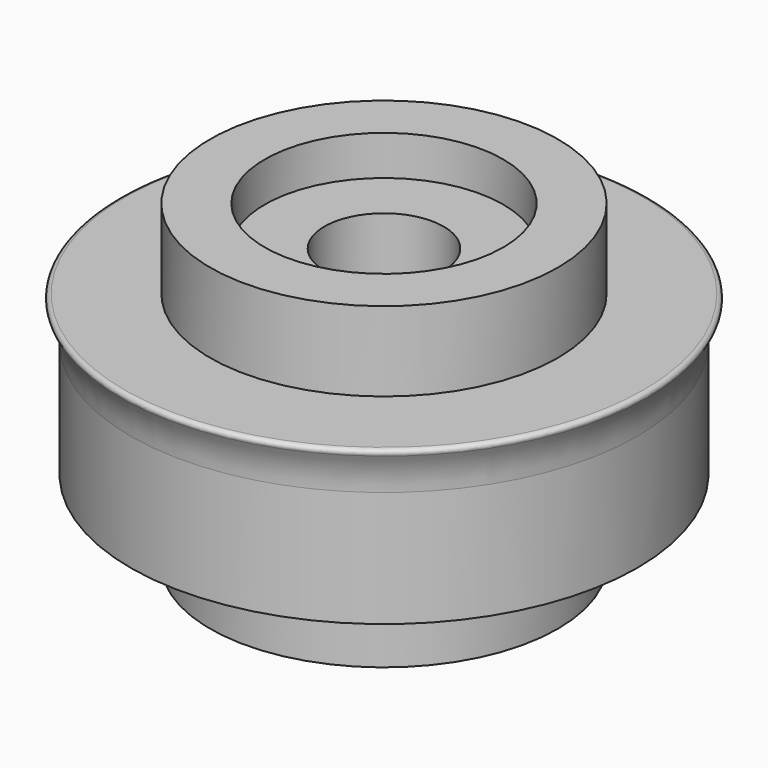
from build123d import *

# Parameters (mm, degrees)
F2_R = 11
F4_R = 0.8


# Not quite as in the source:
# - a fillet or chamfer that OpenCascade refuses, or shapes differently, is made with other operations: its cross-section is extruded or revolved along the edge and cut away or added


with BuildPart() as f1:
    # F0 (on Front) → F1 (revolve)
    with BuildSketch(Plane.XZ):
        Polygon((24, 85.4892928004), (24, 77.4892928004), (12, 77.4892928004), (12, 38.1360072643), (24, 38.1360072643), (24, 21.4892928004), (35, 21.4892928004), (35, 37.4892928004), (51, 37.4892928004), (51, 65.592944622), (51, 69.4892928004), (35, 69.4892928004), (35, 85.4892928004), align=None)
        Polygon((53.7719889283, 69.4892928004), (51, 69.4892928004), (51, 65.592944622), align=None)
    revolve(axis=Axis((0, 0, 48.0438946244), (0, 0, 1)))

    # F2
    f2_edges = [f1.edges().sort_by_distance(p)[0] for p in [
        (-24, 0, 38.136007),
    ]]
    fillet(f2_edges, radius=F2_R)

    # F3: fillet of radius 15 on 1 edges, made by hand


with BuildPart() as f3_tool2:
    # F3_s3 → F3_t4 (revolve)
    with BuildSketch(Plane.XZ):
        with BuildLine():
            ThreePointArc((51, 60.8016097685), (51.7112437374, 65.3657574948), (53.777525929, 69.4970756895))
            Line((53.777525929, 69.4970756895), (51, 65.592944622))
            Line((51, 65.592944622), (51, 60.8016097685))
        make_face()
    revolve(axis=Axis((0, 0, 65.592944622), (0, 0, 1)))

    split(bisect_by=Plane.XY.offset(69.4892928004), keep=Keep.BOTTOM)


with BuildPart() as f1_1:
    add(f1.part)

    # F3_t1: union F3_tool2
    add(f3_tool2.part)

    # F4
    f4_edges = [f1_1.edges().sort_by_distance(p)[0] for p in [
        (-53.771993, 0, 69.489293),
    ]]
    fillet(f4_edges, radius=F4_R)


solid = f1_1.part
